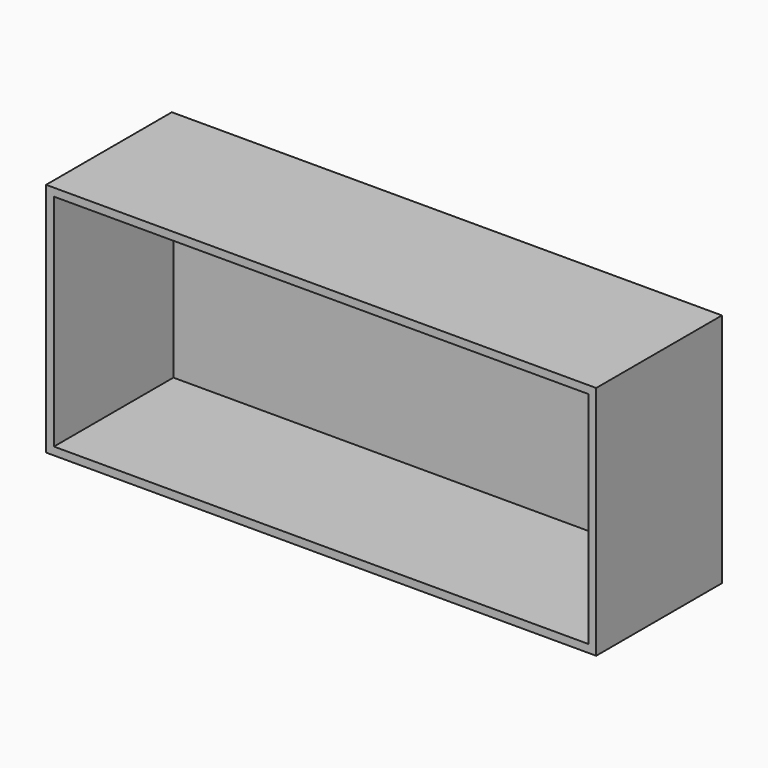
from build123d import *

# Parameters (mm, degrees)
F0_W     = 177.8
F0_H     = 76.2
F1_DEPTH = 50.8
F3_T     = -2.54


# Not quite as in the source:
# - the program builds the solid bodies; features that only make, move or delete a surface that nothing else refers to are left out


with BuildPart() as f1:
    # F0 (on Front) → F1 (new body)
    with BuildSketch(Plane.XZ):
        Rectangle(F0_W, F0_H)
    extrude(amount=F1_DEPTH)

    # F3
    f3_openings = [f1.faces().sort_by_distance(p)[0] for p in [
        (0, -50.8, 0),
    ]]
    offset(amount=F3_T, openings=f3_openings)


solid = f1.part
